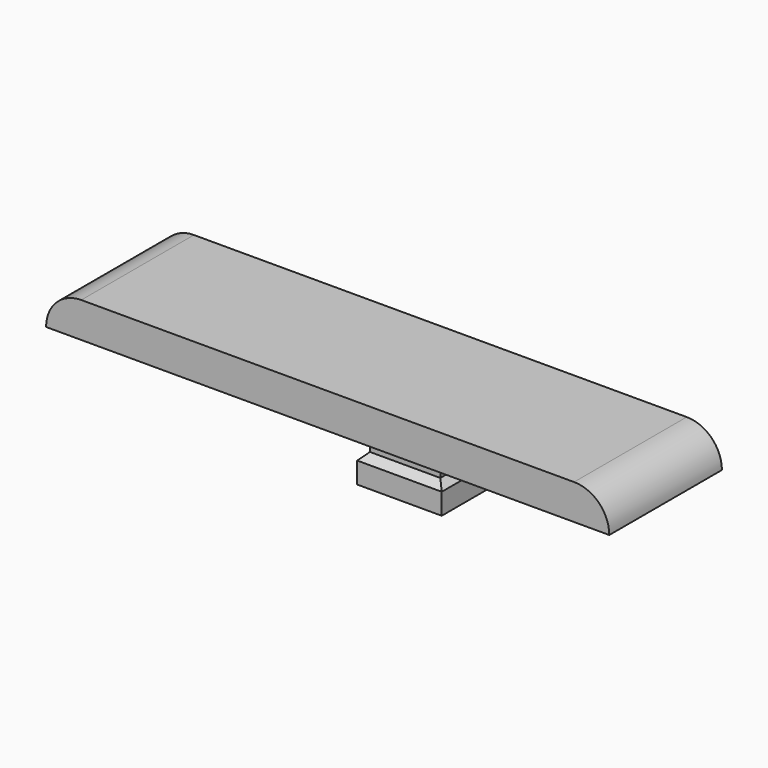
from build123d import *

# Parameters (mm, degrees)
F0_W          = 101.6
F0_H          = 25.4
F0_W_2        = 12.7
F0_H_2        = 12.7
F1_DEPTH      = 6.35
F2_R          = 6.34999
F3_R          = 6.34999
F4_DEPTH      = 3.81
F5_W          = 15.24
F5_H          = 15.24
F5_W_2        = 12.7
F5_H_2        = 12.7
F6_DEPTH      = 6.35
F7_T4_DEPTH   = 28.3041495789
F7_T10_DEPTH  = 28.3041495789
F7_T16_DEPTH  = 28.3041495789
F7_T23_DEPTH  = 28.3041495789
F7_T29_DEPTH  = 28.3041495789
F7_T35_DEPTH  = 28.3041495789
F7_T41_DEPTH  = 28.3041495789
F7_T47_DEPTH  = 28.3041495789
F7_T54_DEPTH  = 28.3041495789
F7_T60_DEPTH  = 28.3041495789
F7_T66_DEPTH  = 28.3041495789
F7_T72_DEPTH  = 28.3041495789
F7_T78_DEPTH  = 28.3041495789
F7_T85_DEPTH  = 28.3041495789
F7_T91_DEPTH  = 28.3041495789
F7_T97_DEPTH  = 28.3041495789
F7_T103_DEPTH = 28.3041495789
F7_T109_DEPTH = 28.3041495789
F7_T116_DEPTH = 28.3041495789
F7_T122_DEPTH = 28.3041495789


# Not quite as in the source:
# - a fillet or chamfer that OpenCascade refuses, or shapes differently, is made with other operations: its cross-section is extruded or revolved along the edge and cut away or added
# - a fillet or chamfer is up to 0.001 mm smaller than in the source, because OpenCascade refuses the exact size


with BuildPart() as f1:
    # F0 (on Top) → F1 (new body)
    with BuildSketch(Plane.XY):
        Rectangle(F0_W, F0_H)
        with Locations((8.89, 0)):
            Rectangle(F0_W_2, F0_H_2, mode=Mode.SUBTRACT)
        with Locations((8.89, 0)):
            Rectangle(F0_W_2, F0_H_2)
    extrude(amount=F1_DEPTH)

    # F2 (radius 6.35 in the source; OpenCascade refuses exactly that, so slightly less here)
    f2_edges = [f1.edges().sort_by_distance(p)[0] for p in [
        (-50.8, 0, 6.35),
    ]]
    fillet(f2_edges, radius=F2_R)

    # F3 (radius 6.35 in the source; OpenCascade refuses exactly that, so slightly less here)
    f3_edges = [f1.edges().sort_by_distance(p)[0] for p in [
        (50.8, 0, 6.35),
    ]]
    fillet(f3_edges, radius=F3_R)

    # F0 (on Top) → F4 (join)
    with BuildSketch(Plane.XY):
        with Locations((8.89, 0)):
            Rectangle(F0_W_2, F0_H_2)
    extrude(amount=-F4_DEPTH)

    # F5 (on face) → F6 (join)
    with BuildSketch(Plane(origin=(0, 0, -3.81), x_dir=(1, 0, 0), z_dir=(0, 0, -1))):
        with Locations((8.89, 0)):
            Rectangle(F5_W, F5_H)
        with Locations((8.89, 0)):
            Rectangle(F5_W_2, F5_H_2, mode=Mode.SUBTRACT)
        with Locations((8.89, 0)):
            Rectangle(F5_W_2, F5_H_2)
    extrude(amount=F6_DEPTH)

    # F7: chamfer of 2.54 on 4 edges, made by hand


with BuildPart() as f7_tool2:
    # F7_s3 → F7_t4 (new body)
    with BuildSketch(Plane.XZ.offset(14.1520747894)):
        Polygon((1.27, -6.35), (3.81, -3.81), (1.27, -3.81), align=None)
    extrude(amount=-F7_T4_DEPTH)

    split(bisect_by=Plane.XZ.offset(6.35), keep=Keep.TOP)

    split(bisect_by=Plane.YZ.offset(2.54), keep=Keep.BOTTOM)


with BuildPart() as f1_1:
    add(f1.part)

    # F7_t1: cut F7_tool2
    add(f7_tool2.part, mode=Mode.SUBTRACT)


with BuildPart() as f7_tool8:
    # F7_s9 → F7_t10 (new body)
    with BuildSketch(Plane.XZ.offset(14.1520747894)):
        Polygon((1.27, -6.35), (3.81, -3.81), (1.27, -3.81), align=None)
    extrude(amount=-F7_T10_DEPTH)

    split(bisect_by=Plane.XZ.offset(6.35), keep=Keep.TOP)

    split(bisect_by=Plane.YZ.offset(2.54), keep=Keep.TOP)


with BuildPart() as f1_2:
    add(f1_1.part)

    # F7_t7: cut F7_tool8
    add(f7_tool8.part, mode=Mode.SUBTRACT)


with BuildPart() as f7_tool14:
    # F7_s15 → F7_t16 (new body)
    with BuildSketch(Plane.XZ.offset(14.1520747894)):
        Polygon((1.27, -6.35), (3.81, -3.81), (1.27, -3.81), align=None)
    extrude(amount=-F7_T16_DEPTH)

    split(bisect_by=Plane.XZ.offset(6.35), keep=Keep.BOTTOM)

    split(bisect_by=Plane.YZ.offset(2.54), keep=Keep.BOTTOM)

    split(bisect_by=Plane.XZ.offset(-6.35), keep=Keep.TOP)


with BuildPart() as f1_3:
    add(f1_2.part)

    # F7_t13: cut F7_tool14
    add(f7_tool14.part, mode=Mode.SUBTRACT)


with BuildPart() as f7_tool21:
    # F7_s22 → F7_t23 (new body)
    with BuildSketch(Plane.XZ.offset(14.1520747894)):
        Polygon((1.27, -6.35), (3.81, -3.81), (1.27, -3.81), align=None)
    extrude(amount=-F7_T23_DEPTH)

    split(bisect_by=Plane.YZ.offset(2.54), keep=Keep.BOTTOM)

    split(bisect_by=Plane.XZ.offset(-6.35), keep=Keep.BOTTOM)


with BuildPart() as f1_4:
    add(f1_3.part)

    # F7_t20: cut F7_tool21
    add(f7_tool21.part, mode=Mode.SUBTRACT)


with BuildPart() as f7_tool27:
    # F7_s28 → F7_t29 (new body)
    with BuildSketch(Plane.XZ.offset(14.1520747894)):
        Polygon((1.27, -6.35), (3.81, -3.81), (1.27, -3.81), align=None)
    extrude(amount=-F7_T29_DEPTH)

    split(bisect_by=Plane.YZ.offset(2.54), keep=Keep.TOP)

    split(bisect_by=Plane.XZ.offset(-6.35), keep=Keep.BOTTOM)


with BuildPart() as f1_5:
    add(f1_4.part)

    # F7_t26: cut F7_tool27
    add(f7_tool27.part, mode=Mode.SUBTRACT)


with BuildPart() as f7_tool33:
    # F7_s34 → F7_t35 (new body)
    with BuildSketch(Plane.YZ.offset(23.0420747894)):
        Polygon((-5.08, -3.81), (-7.62, -6.35), (-7.62, -3.81), align=None)
    extrude(amount=-F7_T35_DEPTH)

    split(bisect_by=Plane.YZ.offset(15.24), keep=Keep.TOP)

    split(bisect_by=Plane.XZ.offset(6.35), keep=Keep.BOTTOM)


with BuildPart() as f1_6:
    add(f1_5.part)

    # F7_t32: cut F7_tool33
    add(f7_tool33.part, mode=Mode.SUBTRACT)


with BuildPart() as f7_tool39:
    # F7_s40 → F7_t41 (new body)
    with BuildSketch(Plane.YZ.offset(23.0420747894)):
        Polygon((-5.08, -3.81), (-7.62, -6.35), (-7.62, -3.81), align=None)
    extrude(amount=-F7_T41_DEPTH)

    split(bisect_by=Plane.YZ.offset(15.24), keep=Keep.TOP)

    split(bisect_by=Plane.XZ.offset(6.35), keep=Keep.TOP)


with BuildPart() as f1_7:
    add(f1_6.part)

    # F7_t38: cut F7_tool39
    add(f7_tool39.part, mode=Mode.SUBTRACT)


with BuildPart() as f7_tool45:
    # F7_s46 → F7_t47 (new body)
    with BuildSketch(Plane.YZ.offset(23.0420747894)):
        Polygon((-5.08, -3.81), (-7.62, -6.35), (-7.62, -3.81), align=None)
    extrude(amount=-F7_T47_DEPTH)

    split(bisect_by=Plane.YZ.offset(15.24), keep=Keep.BOTTOM)

    split(bisect_by=Plane.XZ.offset(6.35), keep=Keep.TOP)

    split(bisect_by=Plane.YZ.offset(2.54), keep=Keep.TOP)


with BuildPart() as f1_8:
    add(f1_7.part)

    # F7_t44: cut F7_tool45
    add(f7_tool45.part, mode=Mode.SUBTRACT)


with BuildPart() as f7_tool52:
    # F7_s53 → F7_t54 (new body)
    with BuildSketch(Plane.YZ.offset(23.0420747894)):
        Polygon((-5.08, -3.81), (-7.62, -6.35), (-7.62, -3.81), align=None)
    extrude(amount=-F7_T54_DEPTH)

    split(bisect_by=Plane.XZ.offset(6.35), keep=Keep.BOTTOM)

    split(bisect_by=Plane.YZ.offset(2.54), keep=Keep.BOTTOM)


with BuildPart() as f1_9:
    add(f1_8.part)

    # F7_t51: cut F7_tool52
    add(f7_tool52.part, mode=Mode.SUBTRACT)


with BuildPart() as f7_tool58:
    # F7_s59 → F7_t60 (new body)
    with BuildSketch(Plane.YZ.offset(23.0420747894)):
        Polygon((-5.08, -3.81), (-7.62, -6.35), (-7.62, -3.81), align=None)
    extrude(amount=-F7_T60_DEPTH)

    split(bisect_by=Plane.XZ.offset(6.35), keep=Keep.TOP)

    split(bisect_by=Plane.YZ.offset(2.54), keep=Keep.BOTTOM)


with BuildPart() as f1_10:
    add(f1_9.part)

    # F7_t57: cut F7_tool58
    add(f7_tool58.part, mode=Mode.SUBTRACT)


with BuildPart() as f7_tool64:
    # F7_s65 → F7_t66 (new body)
    with BuildSketch(Plane.XZ.offset(-14.1520747894)):
        Polygon((16.51, -6.35), (13.97, -3.81), (16.51, -3.81), align=None)
    extrude(amount=F7_T66_DEPTH)

    split(bisect_by=Plane.YZ.offset(15.24), keep=Keep.TOP)

    split(bisect_by=Plane.XZ.offset(-6.35), keep=Keep.BOTTOM)


with BuildPart() as f1_11:
    add(f1_10.part)

    # F7_t63: cut F7_tool64
    add(f7_tool64.part, mode=Mode.SUBTRACT)


with BuildPart() as f7_tool70:
    # F7_s71 → F7_t72 (new body)
    with BuildSketch(Plane.XZ.offset(-14.1520747894)):
        Polygon((16.51, -6.35), (13.97, -3.81), (16.51, -3.81), align=None)
    extrude(amount=F7_T72_DEPTH)

    split(bisect_by=Plane.YZ.offset(15.24), keep=Keep.BOTTOM)

    split(bisect_by=Plane.XZ.offset(-6.35), keep=Keep.BOTTOM)


with BuildPart() as f1_12:
    add(f1_11.part)

    # F7_t69: cut F7_tool70
    add(f7_tool70.part, mode=Mode.SUBTRACT)


with BuildPart() as f7_tool76:
    # F7_s77 → F7_t78 (new body)
    with BuildSketch(Plane.XZ.offset(-14.1520747894)):
        Polygon((16.51, -6.35), (13.97, -3.81), (16.51, -3.81), align=None)
    extrude(amount=F7_T78_DEPTH)

    split(bisect_by=Plane.YZ.offset(15.24), keep=Keep.TOP)

    split(bisect_by=Plane.XZ.offset(6.35), keep=Keep.BOTTOM)

    split(bisect_by=Plane.XZ.offset(-6.35), keep=Keep.TOP)


with BuildPart() as f1_13:
    add(f1_12.part)

    # F7_t75: cut F7_tool76
    add(f7_tool76.part, mode=Mode.SUBTRACT)


with BuildPart() as f7_tool83:
    # F7_s84 → F7_t85 (new body)
    with BuildSketch(Plane.XZ.offset(-14.1520747894)):
        Polygon((16.51, -6.35), (13.97, -3.81), (16.51, -3.81), align=None)
    extrude(amount=F7_T85_DEPTH)

    split(bisect_by=Plane.YZ.offset(15.24), keep=Keep.TOP)

    split(bisect_by=Plane.XZ.offset(6.35), keep=Keep.TOP)


with BuildPart() as f1_14:
    add(f1_13.part)

    # F7_t82: cut F7_tool83
    add(f7_tool83.part, mode=Mode.SUBTRACT)


with BuildPart() as f7_tool89:
    # F7_s90 → F7_t91 (new body)
    with BuildSketch(Plane.XZ.offset(-14.1520747894)):
        Polygon((16.51, -6.35), (13.97, -3.81), (16.51, -3.81), align=None)
    extrude(amount=F7_T91_DEPTH)

    split(bisect_by=Plane.YZ.offset(15.24), keep=Keep.BOTTOM)

    split(bisect_by=Plane.XZ.offset(6.35), keep=Keep.TOP)


with BuildPart() as f1_15:
    add(f1_14.part)

    # F7_t88: cut F7_tool89
    add(f7_tool89.part, mode=Mode.SUBTRACT)


with BuildPart() as f7_tool95:
    # F7_s96 → F7_t97 (new body)
    with BuildSketch(Plane.YZ.offset(-5.2620747894)):
        Polygon((7.62, -6.35), (5.08, -3.81), (7.62, -3.81), align=None)
    extrude(amount=F7_T97_DEPTH)

    split(bisect_by=Plane.YZ.offset(2.54), keep=Keep.BOTTOM)

    split(bisect_by=Plane.XZ.offset(-6.35), keep=Keep.BOTTOM)


with BuildPart() as f1_16:
    add(f1_15.part)

    # F7_t94: cut F7_tool95
    add(f7_tool95.part, mode=Mode.SUBTRACT)


with BuildPart() as f7_tool101:
    # F7_s102 → F7_t103 (new body)
    with BuildSketch(Plane.YZ.offset(-5.2620747894)):
        Polygon((7.62, -6.35), (5.08, -3.81), (7.62, -3.81), align=None)
    extrude(amount=F7_T103_DEPTH)

    split(bisect_by=Plane.YZ.offset(2.54), keep=Keep.BOTTOM)

    split(bisect_by=Plane.XZ.offset(-6.35), keep=Keep.TOP)


with BuildPart() as f1_17:
    add(f1_16.part)

    # F7_t100: cut F7_tool101
    add(f7_tool101.part, mode=Mode.SUBTRACT)


with BuildPart() as f7_tool107:
    # F7_s108 → F7_t109 (new body)
    with BuildSketch(Plane.YZ.offset(-5.2620747894)):
        Polygon((7.62, -6.35), (5.08, -3.81), (7.62, -3.81), align=None)
    extrude(amount=F7_T109_DEPTH)

    split(bisect_by=Plane.YZ.offset(15.24), keep=Keep.BOTTOM)

    split(bisect_by=Plane.YZ.offset(2.54), keep=Keep.TOP)

    split(bisect_by=Plane.XZ.offset(-6.35), keep=Keep.BOTTOM)


with BuildPart() as f1_18:
    add(f1_17.part)

    # F7_t106: cut F7_tool107
    add(f7_tool107.part, mode=Mode.SUBTRACT)


with BuildPart() as f7_tool114:
    # F7_s115 → F7_t116 (new body)
    with BuildSketch(Plane.YZ.offset(-5.2620747894)):
        Polygon((7.62, -6.35), (5.08, -3.81), (7.62, -3.81), align=None)
    extrude(amount=F7_T116_DEPTH)

    split(bisect_by=Plane.YZ.offset(15.24), keep=Keep.TOP)

    split(bisect_by=Plane.XZ.offset(-6.35), keep=Keep.BOTTOM)


with BuildPart() as f1_19:
    add(f1_18.part)

    # F7_t113: cut F7_tool114
    add(f7_tool114.part, mode=Mode.SUBTRACT)


with BuildPart() as f7_tool120:
    # F7_s121 → F7_t122 (new body)
    with BuildSketch(Plane.YZ.offset(-5.2620747894)):
        Polygon((7.62, -6.35), (5.08, -3.81), (7.62, -3.81), align=None)
    extrude(amount=F7_T122_DEPTH)

    split(bisect_by=Plane.YZ.offset(15.24), keep=Keep.TOP)

    split(bisect_by=Plane.XZ.offset(-6.35), keep=Keep.TOP)


with BuildPart() as f1_20:
    add(f1_19.part)

    # F7_t119: cut F7_tool120
    add(f7_tool120.part, mode=Mode.SUBTRACT)


solid = f1_20.part
